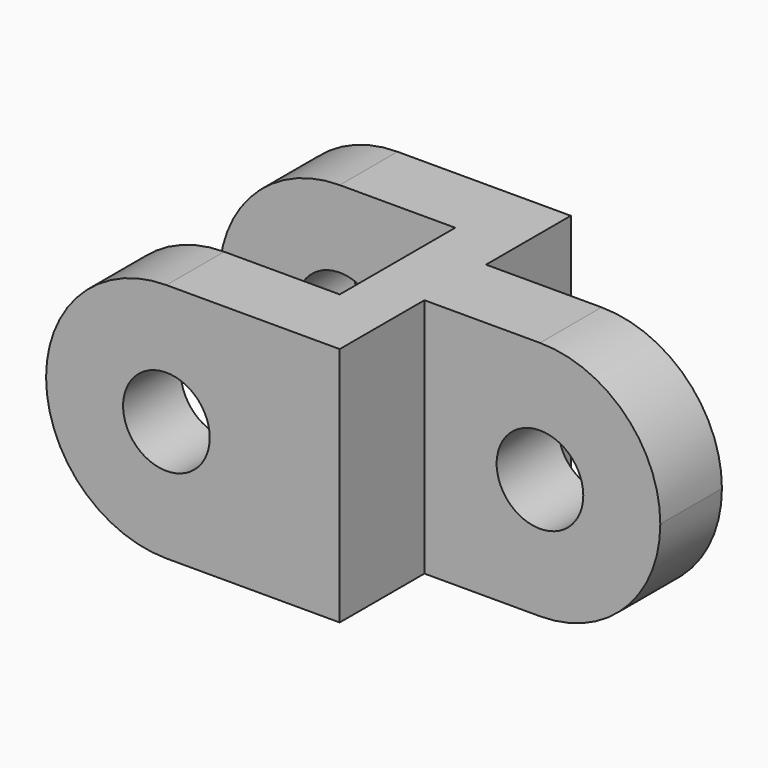
from build123d import *

# Parameters (mm, degrees)
F1_DEPTH = 1270
F2_R     = 634.99999
F3_R     = 228.6
F4_DEPTH = 2540


# Not quite as in the source:
# - a fillet or chamfer is up to 0.001 mm smaller than in the source, because OpenCascade refuses the exact size


with BuildPart() as f1:
    # F0 (on Top) → F1 (new body)
    with BuildSketch(Plane.XY):
        Polygon((700.4859354367, 515.521452381), (-848.9140645633, 515.521452381), (-848.9140645633, 134.521452381), (395.6859354367, 134.521452381), (395.6859354367, -627.478547619), (-848.9140645633, -627.478547619), (-848.9140645633, -1008.478547619), (700.4859354367, -1008.478547619), (700.4859354367, -449.678547619), (1945.0859354367, -449.678547619), (1945.0859354367, -43.278547619), (700.4859354367, -43.278547619), align=None)
    extrude(amount=F1_DEPTH)

    # F2 (radius 635 in the source; OpenCascade refuses exactly that, so slightly less here)
    f2_edges = [f1.edges().sort_by_distance(p)[0] for p in [
        (1945.085935, -246.478548, 1270),
        (1945.085935, -246.478548, 0),
        (-848.914065, -817.978548, 1270),
        (-848.914065, -817.978548, 0),
        (-848.914065, 325.021452, 0),
        (-848.914065, 325.021452, 1270),
    ]]
    fillet(f2_edges, radius=F2_R)

    # F3 (on face) → F4 (cut)
    with BuildSketch(Plane.XZ.offset(1008.478547619)):
        with Locations((-213.9140645633, 635)):
            Circle(F3_R)
        with Locations((1310.0859354367, 635)):
            Circle(F3_R)
    extrude(amount=-F4_DEPTH, mode=Mode.SUBTRACT)


solid = f1.part
